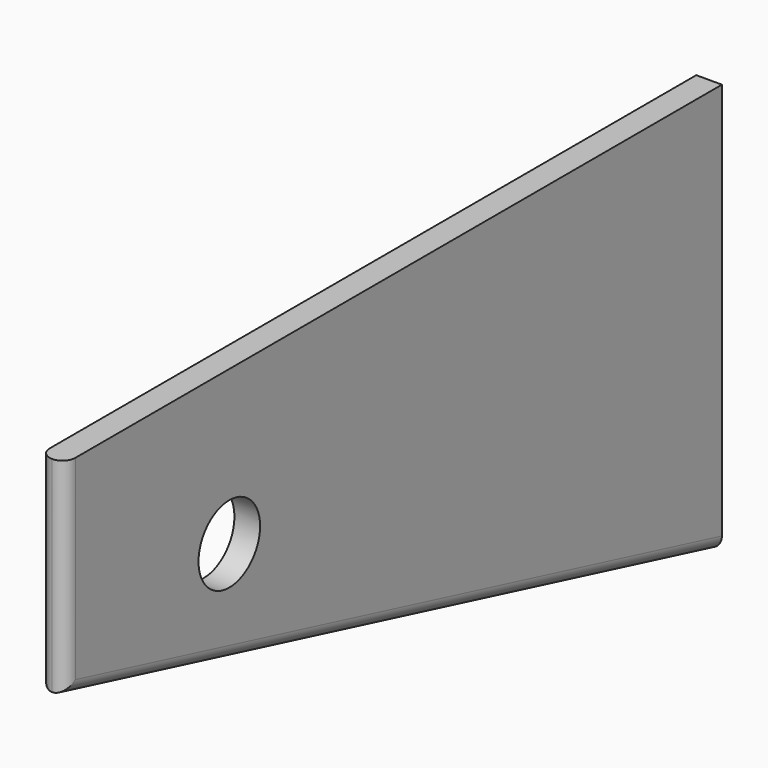
from build123d import *

# Parameters (mm, degrees)
F0_R     = 19.05
F1_DEPTH = 6.35
F2_R     = 6.34999


# Not quite as in the source:
# - a fillet or chamfer is up to 0.001 mm smaller than in the source, because OpenCascade refuses the exact size


with BuildPart() as f1:
    # F0 (on Right) → F1 (new body, symmetric)
    with BuildSketch(Plane.YZ):
        Polygon((406.4, 0), (0, 0), (0, -101.6), (406.4, -203.2), align=None)
        with Locations((101.6, -76.2)):
            Circle(F0_R, mode=Mode.SUBTRACT)
    extrude(amount=F1_DEPTH, both=True)

    # F2 (radius 6.35 in the source; OpenCascade refuses exactly that, so slightly less here)
    f2_edges = [f1.edges().sort_by_distance(p)[0] for p in [
        (-6.35, 203.2, -152.4),
        (6.35, 203.2, -152.4),
        (6.35, 0, -50.8),
        (-6.35, 0, -50.8),
    ]]
    fillet(f2_edges, radius=F2_R)


solid = f1.part
